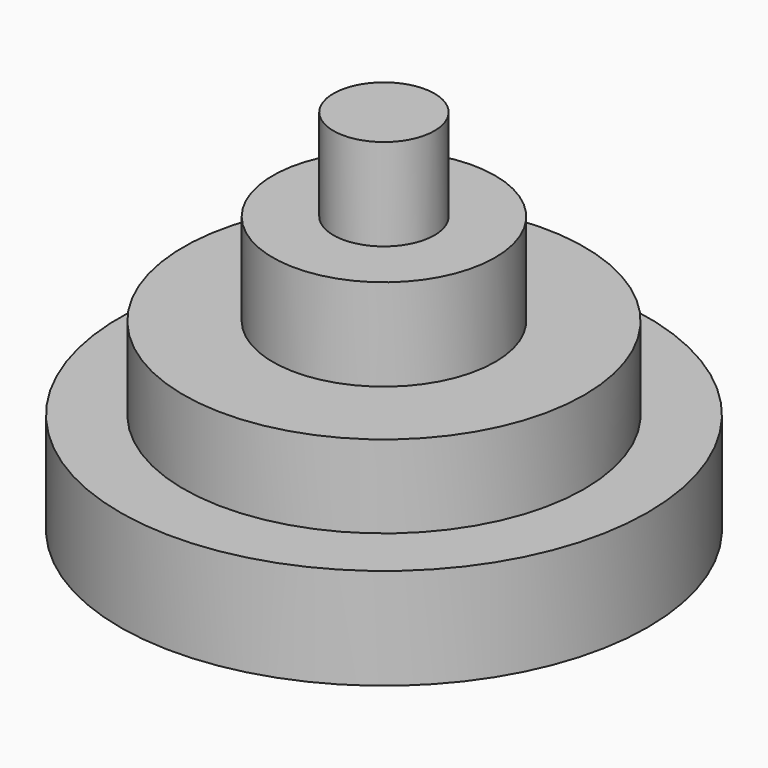
from build123d import *

# Parameters (mm, degrees)
F1_R         = 55.3967717401
F2_DEPTH     = 25.4
F3_TEXT_SIZE = 25.0162918948
F4_DEPTH     = 25.4
F6_DEPTH     = 25.4
F0_R         = 72.9557410348
F7_DEPTH     = 27.94
F8_R         = 30.7189856845
F9_DEPTH     = 25.4
F10_R        = 13.9682325385
F11_DEPTH    = 25.4


# Not quite as in the source:
# - Text() gives the source's letters only with a copy of the font that has no kerning and outlines rounded to 1/6400 em; it was checked with that copy


with BuildPart() as f2:
    # F1 (on Top) → F2 (new body)
    with BuildSketch(Plane.XY):
        Circle(F1_R)
    extrude(amount=F2_DEPTH)

    # F3 (on Top) → F4 (join)
    with BuildSketch(Plane.XY):
        with Locations((-34.7780758804, 0)):
            Text('PEACE', F3_TEXT_SIZE, font='Open Sans', font_style=FontStyle.BOLDITALIC, text_align=(TextAlign.LEFT, TextAlign.BOTTOM))
    extrude(amount=F4_DEPTH)

    # F6 (add): a face of the model
    f6_faces = [f2.faces().sort_by_distance(p)[0] for p in [
        (0, 0, 25.4),
    ]]
    extrude(f6_faces, amount=F6_DEPTH)

    # F0 (on Top) → F7 (join)
    with BuildSketch(Plane.XY):
        Circle(F0_R)
    extrude(amount=F7_DEPTH)

    # F8 (on face) → F9 (join)
    with BuildSketch(Plane.XY.offset(50.8)):
        Circle(F8_R)
    extrude(amount=F9_DEPTH)

    # F10 (on face) → F11 (join)
    with BuildSketch(Plane.XY.offset(76.2)):
        Circle(F10_R)
    extrude(amount=F11_DEPTH)


solid = f2.part
